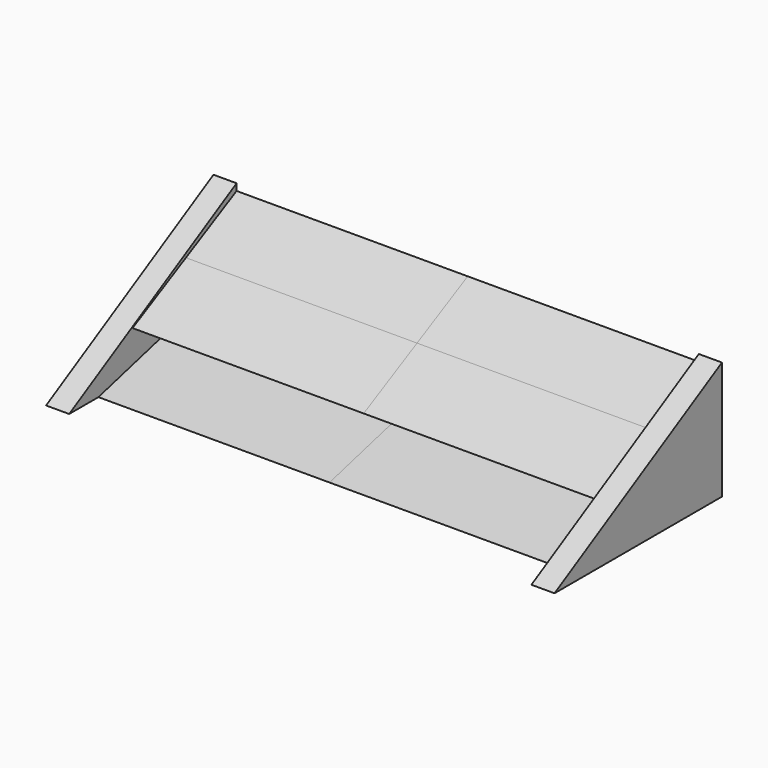
from build123d import *

# Parameters (mm, degrees)
F1_DEPTH = 20
F3_DEPTH = 2


with BuildPart() as f1:
    # F0 (on Right) → F1 (new body)
    with BuildSketch(Plane.YZ):
        Polygon((-70.0796197427, -51.1001968513), (-85.0251993612, -55.0076276596), (-75.5720644497, -55.0076276596), (-75.5589757706, -55.0076276596), (-70.0796197427, -55.0076276596), align=None)
    extrude(amount=F1_DEPTH)


with BuildPart() as f1b:
    # F0 (on Right) → F1, piece 2 (new body)
    with BuildSketch(Plane.YZ):
        Polygon((-81.3316421735, -51.2483594349), (-70.0796197427, -48.3065866685), (-70.0796197427, -45.3729931479), (-75.5589757706, -48.234098685), (-75.5589757706, -48.3106762914), align=None)
        Polygon((-75.5589757706, -48.234098685), (-81.3316421735, -51.2483594349), (-75.5589757706, -48.3106762914), align=None)
    extrude(amount=F1_DEPTH)

    # F2 (on face) → F3 (join)
    with BuildSketch(Plane.YZ.offset(20)):
        Polygon((-88.1861992102, -55.0076276596), (-70.0796197427, -55.0076276596), (-70.0796197427, -44.786806123), align=None)
    extrude(amount=F3_DEPTH)


with BuildPart() as f4_1:
    # F4: instance of F1
    add(f1.part.mirror(Plane.YZ))


with BuildPart() as f4_2:
    # F4: instance of F1b
    add(f1b.part.mirror(Plane.YZ))


solid = Compound([f1.part, f1b.part, f4_1.part, f4_2.part])
